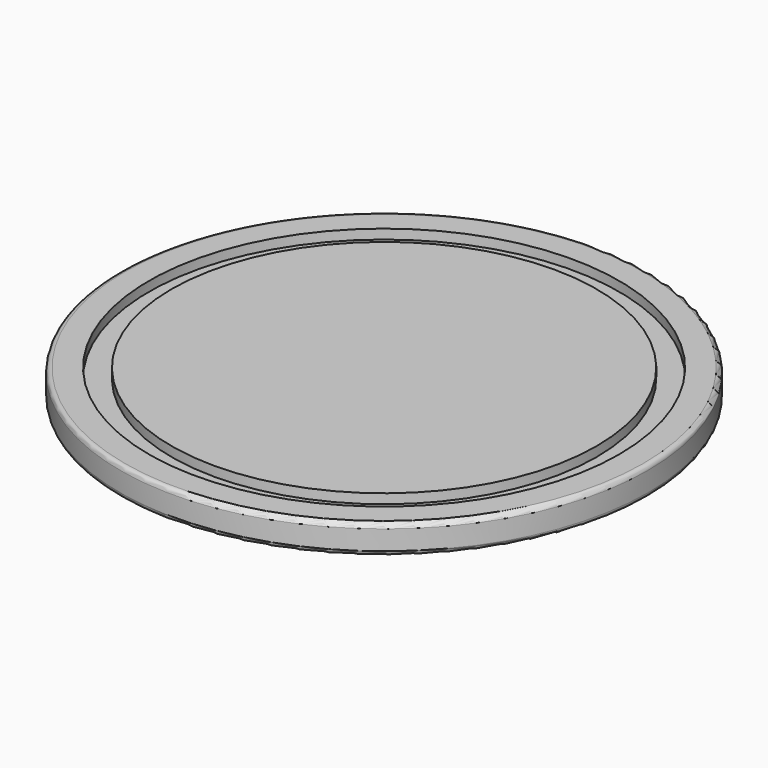
from build123d import *

# Parameters (mm, degrees)
F0_R     = 23.368
F1_DEPTH = 1.0583333333
F0_R_2   = 29.0195
F0_R_3   = 25.8445
F2_R     = 29.0195
F2_R_2   = 23.368
F3_DEPTH = 1.0583333333
F4_R     = 29.0195
F4_R_2   = 25.8445
F4_R_3   = 23.368
F5_DEPTH = 1.0583333333
F6_R     = 0.508


with BuildPart() as f1:
    # F0 (on Top) → F1 (new body)
    with BuildSketch(Plane.XY):
        Circle(F0_R)
    extrude(amount=F1_DEPTH)



with BuildPart() as f1b:
    # F0 (on Top) → F1, piece 2 (new body)
    with BuildSketch(Plane.XY):
        Circle(F0_R_2)
        Circle(F0_R_3, mode=Mode.SUBTRACT)
    extrude(amount=F1_DEPTH)


with BuildPart() as f1_1:
    add(f1.part)

    add(f1b.part)  # F3 merges F1b
    # F2 (on face) → F3 (join)
    with BuildSketch(Plane(origin=(0, 0, 0), x_dir=(1, 0, 0), z_dir=(0, 0, -1))):
        Circle(F2_R)
        Circle(F2_R_2, mode=Mode.SUBTRACT)
        Circle(F2_R_2)
    extrude(amount=F3_DEPTH)

    # F4 (on face) → F5 (join)
    with BuildSketch(Plane(origin=(0, 0, -1.0583333333), x_dir=(1, 0, 0), z_dir=(0, 0, -1))):
        Circle(F4_R)
        Circle(F4_R_2, mode=Mode.SUBTRACT)
        Circle(F4_R_3)
    extrude(amount=F5_DEPTH)

    # F6
    f6_edges = [f1_1.edges().sort_by_distance(p)[0] for p in [
        (-29.0195, 0, -2.116667),
        (-29.0195, 0, 1.058333),
    ]]
    fillet(f6_edges, radius=F6_R)


solid = f1_1.part
